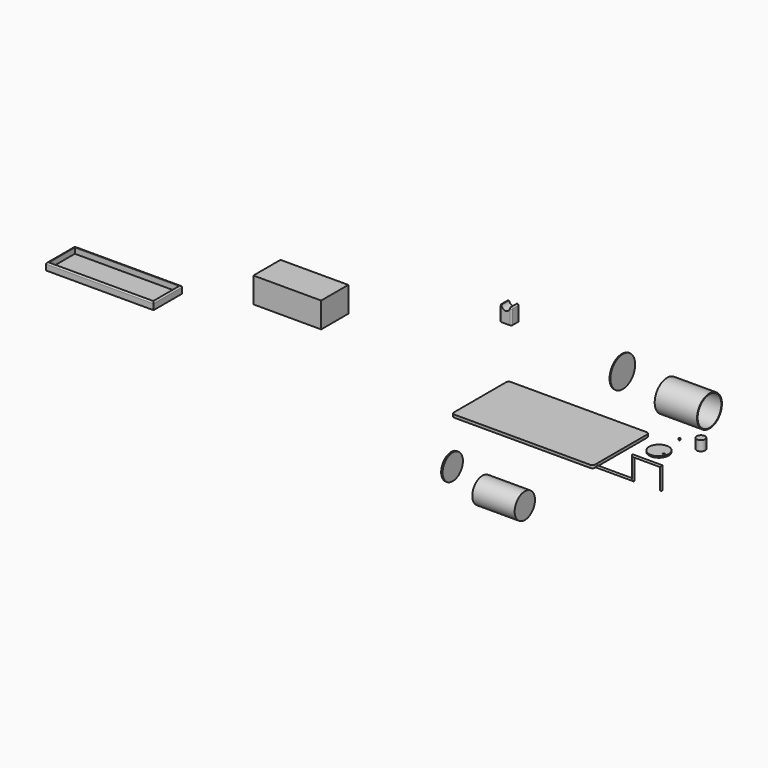
from build123d import *

# Parameters (mm, degrees)
F0_W      = 500
F0_H      = 250
F1_DEPTH  = 10
F2_R      = 55
F3_DEPTH  = 150
F4_T      = -2.5
F5_R      = 10
F6_R      = 54.75
F7_DEPTH  = 3
F9_R      = 3.5
F11_R     = 35
F12_DEPTH = 5
F13_R     = 15
F14_DEPTH = 35
F15_R     = 2.5
F16_DEPTH = 5
F17_W     = 40
F17_H     = 35
F18_DEPTH = 55
F20_DEPTH = 40
F21_R     = 4.999
F23_D     = 7
F24_W     = 240
F24_H     = 120
F25_DEPTH = 90
F26_R     = 45
F27_DEPTH = 150
F28_T     = -2.5
F29_R     = 45
F30_DEPTH = 5
F31_W     = 380.425453186
F31_H     = 126.8084421754
F32_DEPTH = 25
F33_R     = 5
F34_T     = -2.5


# Not quite as in the source:
# - a fillet or chamfer is up to 0.001 mm smaller than in the source, because OpenCascade refuses the exact size
# - a shell that OpenCascade refuses in one call is made with other operations: the cavity is built on its own and cut out


with BuildPart() as f1:
    # F0 (on Top) → F1 (new body)
    with BuildSketch(Plane.XY):
        with Locations((-177.4380993843, 106.5403278917)):
            Rectangle(F0_W, F0_H)
    extrude(amount=F1_DEPTH)

    # F5
    f5_edges = [f1.edges().sort_by_distance(p)[0] for p in [
        (72.561901, 231.540328, 5),
        (-427.438099, 231.540328, 5),
        (-427.438099, -18.459672, 5),
        (72.561901, -18.459672, 5),
    ]]
    fillet(f5_edges, radius=F5_R)


with BuildPart() as f3:
    # F2 (on Right) → F3 (new body)
    with BuildSketch(Plane.YZ):
        with Locations((400.5251824856, 35.6430858374)):
            Circle(F2_R)
    extrude(amount=F3_DEPTH)

    # F4
    f4_openings = [f3.faces().sort_by_distance(p)[0] for p in [
        (150, 400.525182, 35.643086),
    ]]
    offset(amount=F4_T, openings=f4_openings)


with BuildPart() as f7:
    # F6 (on Right) → F7 (new body)
    with BuildSketch(Plane.YZ):
        with Locations((200.5351930857, 191.765576601)):
            Circle(F6_R)
    extrude(amount=F7_DEPTH)


with BuildPart() as f10:
    # F10: sweep along a path in F8
    with BuildLine(Plane.XZ) as f10_path:
        Line((0, 0), (200, 0))
        Line((200, 0), (200, 75))
        Line((200, 75), (300, 75))
        Line((300, 75), (300, 0))
    # F9 (on Right) → F10 (sweep)
    with BuildSketch(Plane.YZ):
        Circle(F9_R)
    sweep(path=f10_path.line, transition=Transition.RIGHT)


with BuildPart() as f12:
    # F11 (on Top) → F12 (new body)
    with BuildSketch(Plane.XY):
        with Locations((151.3125747442, 175.1156896353)):
            Circle(F11_R)
    extrude(amount=F12_DEPTH)

    # F23 (through all)
    with Locations(Plane(origin=(0, 0, 0), x_dir=(1, 0, 0), z_dir=(0, 0, -1))):
        with Locations((175.1386225224, -167.4195230007)):
            Hole(F23_D / 2)


with BuildPart() as f14:
    # F13 (on Top) → F14 (new body)
    with BuildSketch(Plane.XY):
        with Locations((230.6227236986, 261.7385685444)):
            Circle(F13_R)
    extrude(amount=F14_DEPTH)


with BuildPart() as f16:
    # F15 (on Top) → F16 (new body)
    with BuildSketch(Plane.XY):
        with Locations((150.4363566637, 267.1612799168)):
            Circle(F15_R)
    extrude(amount=F16_DEPTH)


with BuildPart() as f18:
    # F17 (on Top) → F18 (new body)
    with BuildSketch(Plane.XY):
        with Locations((-659.1219115257, 527.3338127136)):
            Rectangle(F17_W, F17_H)
    extrude(amount=F18_DEPTH)

    # F19 (on face) → F20 (cut)
    with BuildSketch(Plane.XZ.offset(-509.8338127136)):
        with BuildLine():
            Line((-644.1229029035, 55), (-674.1219115257, 55))
            ThreePointArc((-674.1219115257, 55), (-659.1224072146, 39.8780556624), (-644.1229029035, 55))
        make_face()
    extrude(amount=-F20_DEPTH, mode=Mode.SUBTRACT)

    # F21 (radius 5 in the source; OpenCascade refuses exactly that, so slightly less here)
    f21_edges = [f18.edges().sort_by_distance(p)[0] for p in [
        (-679.121912, 527.333813, 55),
        (-676.621912, 509.833813, 55),
        (-679.121912, 509.833813, 27.5),
        (-639.121912, 509.833813, 27.5),
        (-641.622407, 509.833813, 55),
        (-639.121912, 544.833813, 27.5),
        (-639.121912, 527.333813, 55),
        (-641.622407, 544.833813, 55),
        (-676.621912, 544.833813, 55),
        (-679.121912, 544.833813, 27.5),
    ]]
    fillet(f21_edges, radius=F21_R)


with BuildPart() as f25:
    # F24 (on Top) → F25 (new body)
    with BuildSketch(Plane.XY):
        with Locations((-1156.1287093163, 224.6164506674)):
            Rectangle(F24_W, F24_H)
    extrude(amount=F25_DEPTH)


with BuildPart() as f27:
    # F26 (on Right) → F27 (new body)
    with BuildSketch(Plane.YZ):
        with Locations((-416.7462587357, 72.744615376)):
            Circle(F26_R)
    extrude(amount=F27_DEPTH)

    # F28
    f28_openings = [f27.faces().sort_by_distance(p)[0] for p in [
        (0, -416.746259, 72.744615),
    ]]
    offset(amount=F28_T, openings=f28_openings)


with BuildPart() as f30:
    # F29 (on Right) → F30 (new body)
    with BuildSketch(Plane.YZ):
        with Locations((-554.5350313187, 202.644765377)):
            Circle(F29_R)
    extrude(amount=F30_DEPTH)


with BuildPart() as f32:
    # F31 (on Top) → F32 (new body)
    with BuildSketch(Plane.XY):
        with Locations((-1660.0656509399, 28.3213891089)):
            Rectangle(F31_W, F31_H)
    extrude(amount=F32_DEPTH)

    # F33
    f33_edges = [f32.edges().sort_by_distance(p)[0] for p in [
        (-1660.065651, -35.082832, 25),
        (-1469.852924, 28.321389, 25),
        (-1660.065651, 91.72561, 25),
        (-1850.278378, 28.321389, 25),
    ]]
    fillet(f33_edges, radius=F33_R)

    # F34: a shell. OpenCascade refuses it in one call, so the cavity is built on its own and cut out:
    # the body offset inwards by the wall thickness, plus a prism from it out through each open face.
    f34_core = offset(f32.part, amount=F34_T, mode=Mode.PRIVATE)
    f34_exits = [f34_core.faces().sort_by_distance(p)[0] for p in [
        (-1660.065651, 28.321389, 22.5),
    ]]
    add(f34_core, mode=Mode.SUBTRACT)
    extrude(f34_exits, amount=-F34_T, mode=Mode.SUBTRACT)


solid = Compound([f1.part, f3.part, f7.part, f10.part, f12.part, f14.part, f16.part, f18.part, f25.part, f27.part, f30.part, f32.part])
